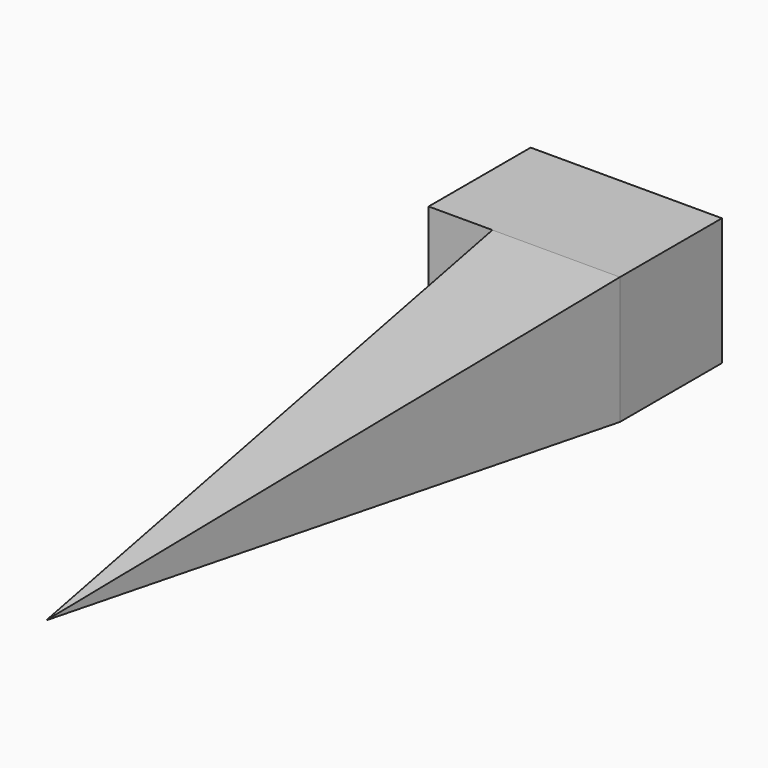
from build123d import *

# Parameters (mm, degrees)
F0_W     = 10
F0_H     = 50
F0_H_2   = 10
F0_W_2   = 5
F1_DEPTH = 10
F2_SIZE2 = 49.99999
F2_SIZE  = 4.99999


# Not quite as in the source:
# - a fillet or chamfer is up to 0.001 mm smaller than in the source, because OpenCascade refuses the exact size


with BuildPart() as f1:
    # F0 (on Top) → F1 (new body)
    with BuildSketch(Plane.XY):
        with Locations((-5, -25)):
            Rectangle(F0_W, F0_H)
        with Locations((-5, 5)):
            Rectangle(F0_W, F0_H_2)
        with Locations((-12.5, 5)):
            Rectangle(F0_W_2, F0_H_2)
    extrude(amount=F1_DEPTH)

    # F2 (size 5 and 50 in the source; OpenCascade refuses exactly that, so slightly less here)
    f2_edges = [f1.edges().sort_by_distance(p)[0] for p in [
        (-5, -50, 10),
        (-10, -50, 5),
        (-5, -50, 0),
        (0, -50, 5),
    ]]
    f2_side = f1.faces().sort_by_distance((-5, -50, 5))[0]
    chamfer(f2_edges, length=F2_SIZE, length2=F2_SIZE2, reference=f2_side)


solid = f1.part
